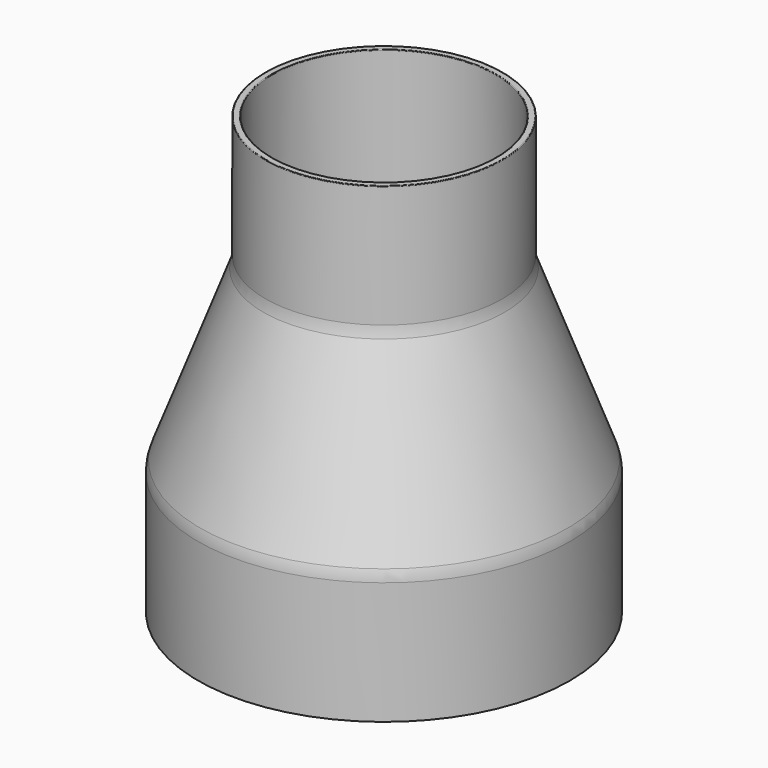
from build123d import *

# Parameters (mm, degrees)
F2_R = 5
F3_R = 0.1


with BuildPart() as f1:
    # F0 (on Front) → F1 (revolve)
    with BuildSketch(Plane.XZ):
        Polygon((-29, 20), (-29, 0), (-28, 0), (-28, 19.8192848565), (-17.5, 47.9217758492), (-17.5, 68.1024909928), (-18.5, 68.1024909928), (-18.5, 48.1024909928), align=None)
    revolve(axis=Axis((0, 0, 23.4480407089), (0, 0, 1)))

    # F2
    f2_edges = [f1.edges().sort_by_distance(p)[0] for p in [
        (29, 0, 20),
        (18.5, 0, 48.102491),
    ]]
    fillet(f2_edges, radius=F2_R)

    # F3
    f3_edges = [f1.edges().sort_by_distance(p)[0] for p in [
        (17.5, 0, 68.102491),
        (18.5, 0, 68.102491),
    ]]
    fillet(f3_edges, radius=F3_R)


solid = f1.part
